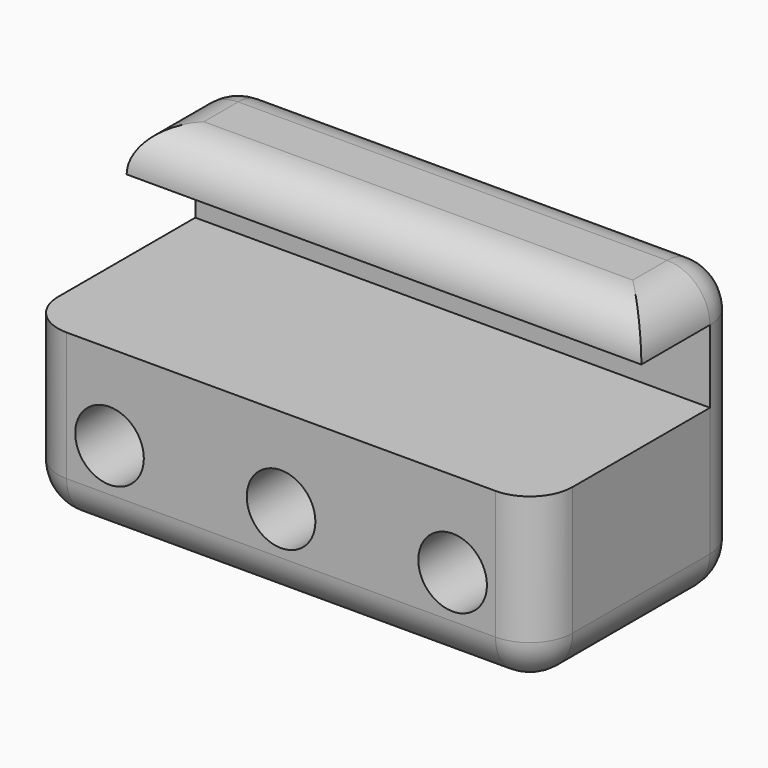
from build123d import *

# Parameters (mm, degrees)
F0_W     = 60
F0_H     = 20
F1_DEPTH = 30
F2_W     = 60
F2_H     = 8.5
F3_DEPTH = 5
F4_W     = 60
F4_H     = 5
F5_DEPTH = 15
F6_R     = 4
F7_DEPTH = 30.001
F8_R     = 4.99999


# Not quite as in the source:
# - a fillet or chamfer is up to 0.001 mm smaller than in the source, because OpenCascade refuses the exact size


with BuildPart() as f1:
    # F0 (on Front) → F1 (new body)
    with BuildSketch(Plane.XZ):
        with Locations((0, -10)):
            Rectangle(F0_W, F0_H)
    extrude(amount=F1_DEPTH)

    # F2 (on Front) → F3 (join)
    with BuildSketch(Plane.XZ):
        with Locations((0, 4.25)):
            Rectangle(F2_W, F2_H)
    extrude(amount=F3_DEPTH)

    # F4 (on Front) → F5 (join)
    with BuildSketch(Plane.XZ):
        with Locations((0, 11)):
            Rectangle(F4_W, F4_H)
    extrude(amount=F5_DEPTH)

    # F6 (on Front) → F7 (cut, through all)
    with BuildSketch(Plane.XZ):
        with Locations((-20, -10)):
            Circle(F6_R)
        with Locations((0, -10)):
            Circle(F6_R)
        with Locations((20, -10)):
            Circle(F6_R)
    extrude(amount=F7_DEPTH, mode=Mode.SUBTRACT)

    # F8 (radius 5 in the source; OpenCascade refuses exactly that, so slightly less here)
    f8_edges = [f1.edges().sort_by_distance(p)[0] for p in [
        (30, -15, -20),
        (30, -30, -10),
        (30, -7.5, 13.5),
        (0, 0, 13.5),
        (0, 0, -20),
        (-30, -15, -20),
        (0, -30, -20),
        (-30, -30, -10),
        (-30, -7.5, 13.5),
        (-30, 0, -3.25),
        (0, -15, 13.5),
        (30, 0, -3.25),
    ]]
    fillet(f8_edges, radius=F8_R)


solid = f1.part
